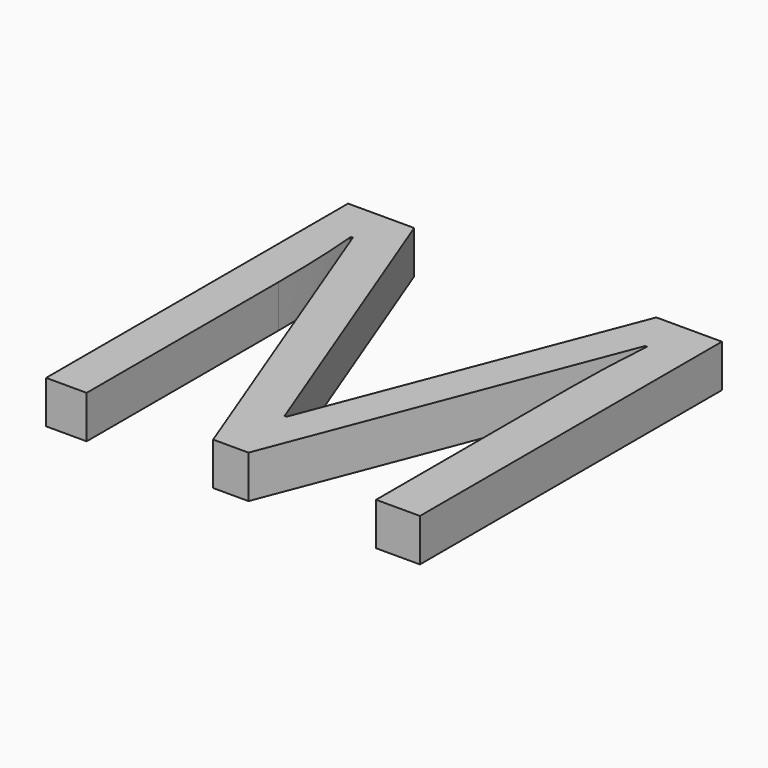
from build123d import *

# Parameters (mm, degrees)
F0_TEXT_SIZE = 9.4365890307
F1_DEPTH     = 0.762


# Not quite as in the source:
# - Text() gives the source's letters only with a copy of the font that has no kerning and outlines rounded to 1/6400 em; it was checked with that copy


with BuildPart() as f1:
    # F0 (on Top) → F1 (new body)
    with BuildSketch(Plane.XY):
        with Locations((-8.2098324567, 0)):
            Text('M', F0_TEXT_SIZE, font='Open Sans', text_align=(TextAlign.LEFT, TextAlign.BOTTOM))
    extrude(amount=F1_DEPTH)


solid = f1.part
